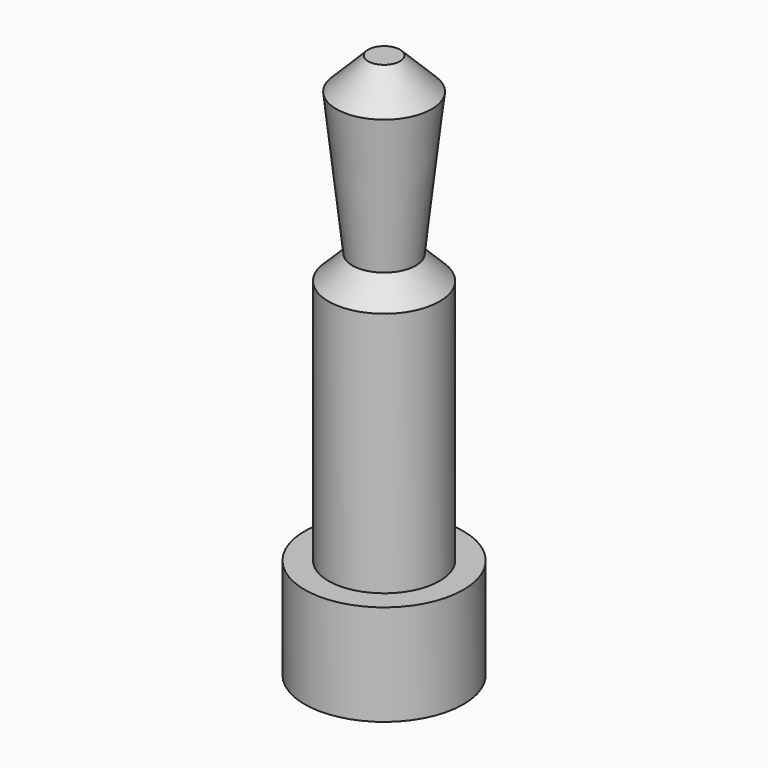
from build123d import *

# Parameters (mm, degrees)
F0_R      = 2.5
F1_DEPTH  = 3.175
F2_R      = 1.75
F3_DEPTH  = 8.5
F4_SIZE   = 0.75
F5_R      = 1
F7_R      = 1.5
F9_R      = 1.5
F10_DEPTH = 1
F11_SIZE  = 0.99999


# Not quite as in the source:
# - a fillet or chamfer is up to 0.001 mm smaller than in the source, because OpenCascade refuses the exact size


with BuildPart() as f1:
    # F0 (on Top) → F1 (new body)
    with BuildSketch(Plane.XY):
        Circle(F0_R)
    extrude(amount=F1_DEPTH)

    # F2 (on face) → F3 (join)
    with BuildSketch(Plane.XY.offset(3.175)):
        Circle(F2_R)
    extrude(amount=F3_DEPTH)

    # F4
    f4_edges = [f1.edges().sort_by_distance(p)[0] for p in [
        (-1.75, 0, 11.675),
    ]]
    chamfer(f4_edges, length=F4_SIZE)

    # F5 (on face) → F8 section 0
    with BuildSketch(Plane.XY.offset(11.675)):
        Circle(F5_R)
    # F7 (on offset) → F8 section 1
    with BuildSketch(Plane.XY.offset(16.175)):
        Circle(F7_R)
    loft()

    # F9 (on face) → F10 (join)
    with BuildSketch(Plane.XY.offset(16.175)):
        Circle(F9_R)
    extrude(amount=F10_DEPTH)

    # F11 (size 1 in the source; OpenCascade refuses exactly that, so slightly less here)
    f11_edges = [f1.edges().sort_by_distance(p)[0] for p in [
        (-1.5, 0, 17.175),
    ]]
    chamfer(f11_edges, length=F11_SIZE)


solid = f1.part
